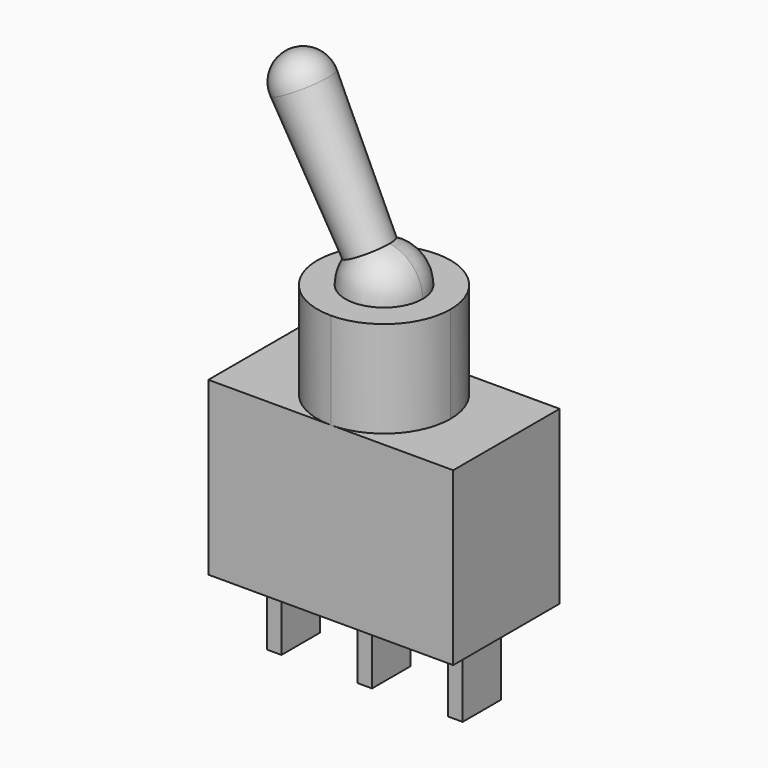
from build123d import *
from build123d import SkipClean  # not in build123d's __all__

# Parameters (mm, degrees)
F0_W     = 12.7
F0_H     = 6.9
F1_DEPTH = 8.9
F3_DEPTH = 5
F8_W     = 0.76
F8_H     = 2.5
F9_DEPTH = 3.9


with BuildPart() as f1:
    # F0 (on Top) → F1 (new body)
    with BuildSketch(Plane.XY):
        with Locations((6.35, 0)):
            Rectangle(F0_W, F0_H)
    extrude(amount=F1_DEPTH)

    # F2 (on face) → F3 (join)
    with BuildSketch(Plane.XY.offset(8.9)):
        with BuildLine():
            ThreePointArc((6.35, -3.45), (8.7895183951, -2.4395183951), (9.8, 0))
            ThreePointArc((9.8, 0), (8.7895183951, 2.4395183951), (6.35, 3.45))
            ThreePointArc((6.35, 3.45), (2.9, 0), (6.35, -3.45))
        make_face()
    extrude(amount=F3_DEPTH)

    # F4 (on Front) → F5 (revolve)
    with BuildSketch(Plane.XZ):
        with BuildLine():
            Line((0.9029362769, 21.0829250706), (5.05, 13.9))
            Line((5.05, 13.9), (6.35, 13.9))
            Line((6.35, 13.9), (1.4796313262, 23.0890972887))
            ThreePointArc((1.4796313262, 23.0890972887), (0.7651079647, 22.2085198521), (0.9029362769, 21.0829250706))
        make_face()
    revolve(axis=Axis((3.9148156631, 0, 18.4945486443), (0.4683046802, 0, -0.883567047)))

    # F6 (on Front) → F7 (revolve)
    with BuildSketch(Plane.XZ):
        with BuildLine():
            ThreePointArc((8.35, 13.9), (6.35, 15.9), (4.35, 13.9))
            Line((4.35, 13.9), (8.35, 13.9))
        make_face()
    with SkipClean():  # cleaning this boolean's faces spoils the solid; the shape is the same uncleaned
        revolve(axis=Axis((6.35, 0, 13.9), (1, 0, 0)))

    # F8 (on Top) → F9 (join)
    with BuildSketch(Plane.XY):
        with Locations((1.65, 0)):
            Rectangle(F8_W, F8_H)
        with Locations((6.35, 0)):
            Rectangle(F8_W, F8_H)
        with Locations((11.05, 0)):
            Rectangle(F8_W, F8_H)
    with SkipClean():  # cleaning this boolean's faces spoils the solid; the shape is the same uncleaned
        extrude(amount=-F9_DEPTH)


solid = f1.part
